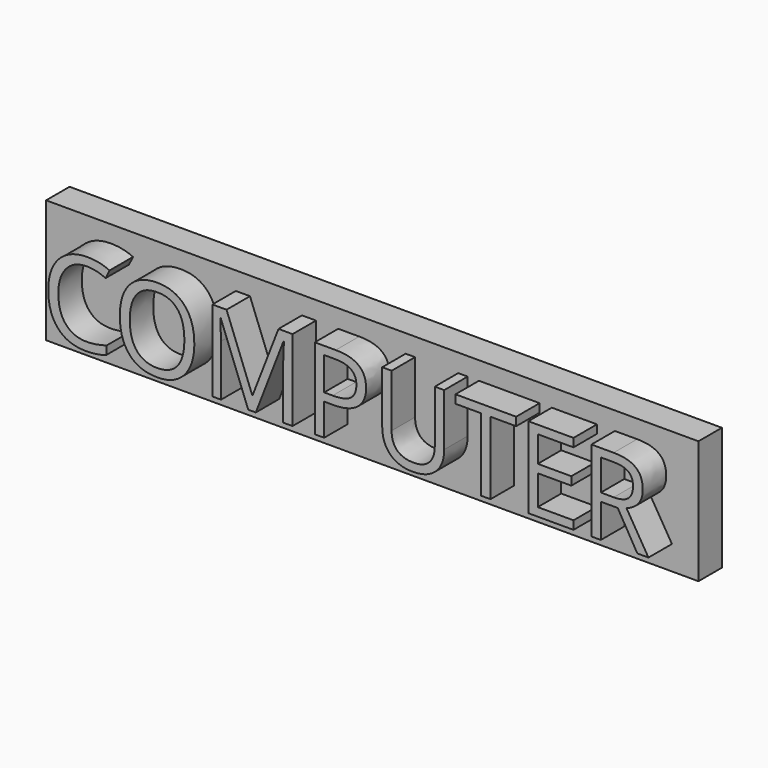
from build123d import *

# Parameters (mm, degrees)
F0_W         = 555.7867884636
F0_H         = 104.9748882651
F2_DEPTH     = 25
F1_TEXT_SIZE = 96.6257752023
F3_DEPTH     = 25


# Not quite as in the source:
# - Text() gives the source's letters only with a copy of the font that has no kerning and outlines rounded to 1/6400 em; it was checked with that copy


with BuildPart() as f2:
    # F0 (on Front) → F2 (new body)
    with BuildSketch(Plane.XZ):
        with Locations((277.8933942318, 52.4874441326)):
            Rectangle(F0_W, F0_H)
    extrude(amount=-F2_DEPTH)

    # F1 (on Front) → F3 (join)
    with BuildSketch(Plane.XZ):
        with Locations((15.9707982093, 20.5883812159)):
            Text('COMPUTER', F1_TEXT_SIZE, font='Open Sans', text_align=(TextAlign.LEFT, TextAlign.BOTTOM))
    extrude(amount=F3_DEPTH)


solid = f2.part
